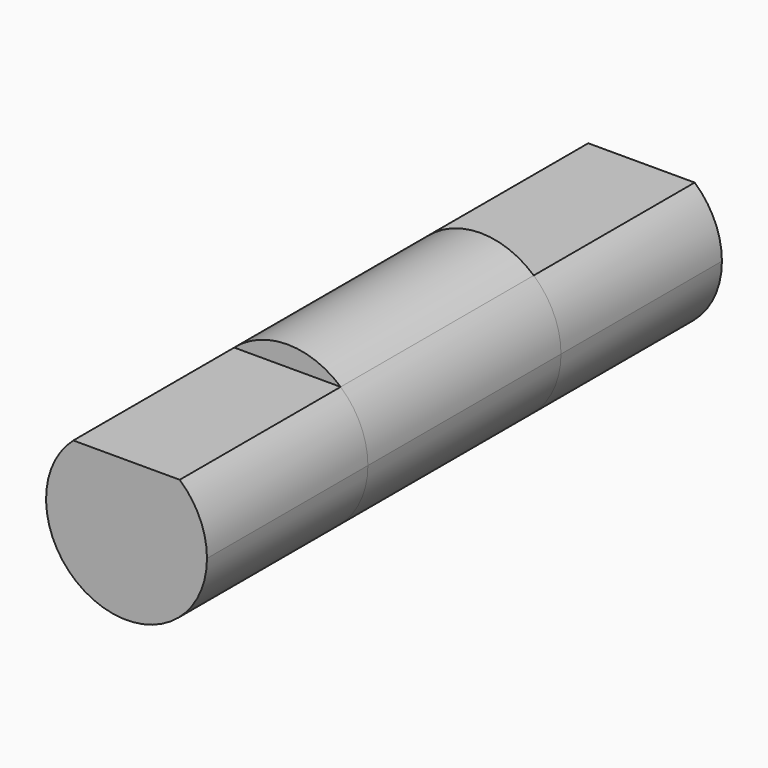
from build123d import *
from build123d import SkipClean  # not in build123d's __all__

# Parameters (mm, degrees)
F1_DEPTH = 16
F3_START = -5
F2_R     = 2
F3_DEPTH = 6


with BuildPart() as f1:
    # F0 (on Front) → F1 (new body)
    with BuildSketch(Plane.XZ):
        with BuildLine():
            ThreePointArc((-1.3228756555, 1.5), (-0.8228756555, -1.8228756555), (2, 0))
            ThreePointArc((2, 0), (1.8228756555, 0.8228756555), (1.3228756555, 1.5))
            Line((1.3228756555, 1.5), (-1.3228756555, 1.5))
        make_face()
    extrude(amount=F1_DEPTH)

    # F2 (on face) → F3 (join)
    with BuildSketch(Plane.XZ.offset(16).offset(F3_START)):
        Circle(F2_R)
    with SkipClean():  # cleaning this boolean's faces spoils the solid; the shape is the same uncleaned
        extrude(amount=-F3_DEPTH)


solid = f1.part
